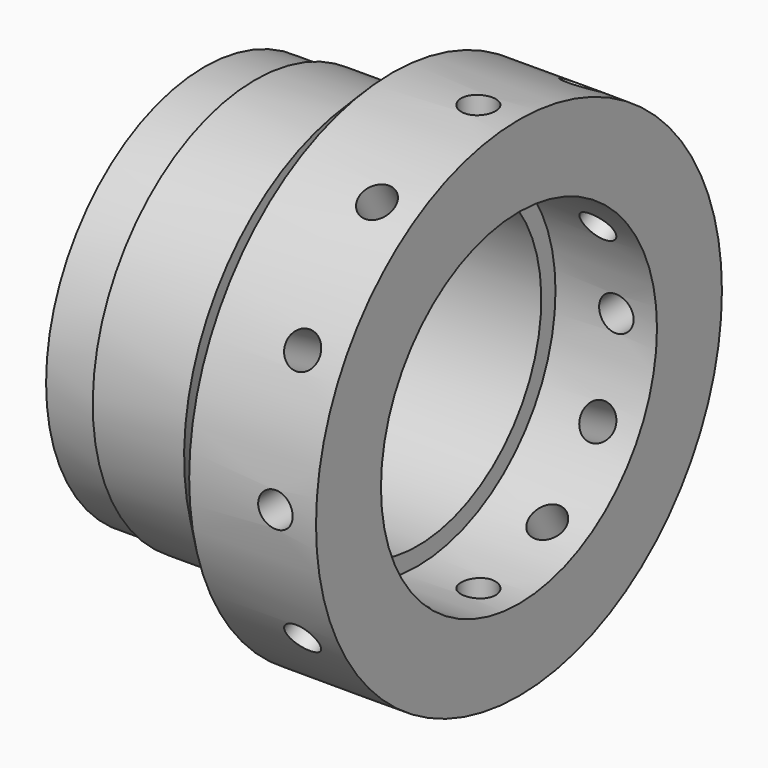
from build123d import *

# Parameters (mm, degrees)
F2_SIZE         = 5
F3_R            = 3.4
F4_DEPTH        = 50.001
F4_COPIES_COUNT = 12


# Not quite as in the source:
# - a pattern or mirror of a feature is missing from the dataset's text; its kind, count and spacing are read off the source's solid


with BuildPart() as f1:
    # F0 (on Front) → F1 (revolve)
    with BuildSketch(Plane.XZ):
        Polygon((0, 39), (0, 30.5), (42, 30.5), (42, 34), (62, 34), (62, 50), (32, 50), (32, 40), (10, 40), (10, 39), align=None)
    revolve(axis=Axis((20.1939043789, 0, 0), (1, 0, 0)))

    # F2
    f2_edges = [f1.edges().sort_by_distance(p)[0] for p in [
        (32, 0, -50),
    ]]
    chamfer(f2_edges, length=F2_SIZE)

    # F3 (on Top) → F4 (cut, through all)
    with BuildSketch(Plane.XY):
        with Locations((54, 0)):
            Circle(F3_R)
    f4 = extrude(amount=-F4_DEPTH, mode=Mode.SUBTRACT)

    # F4_copies: F4 ×12 about axis
    f4_copies_axis = Axis((0, 0, 0), (1, 0, 0))
    for i in range(1, F4_COPIES_COUNT):
        add(f4.rotate(f4_copies_axis, i * 360 / F4_COPIES_COUNT), mode=Mode.SUBTRACT)


solid = f1.part
